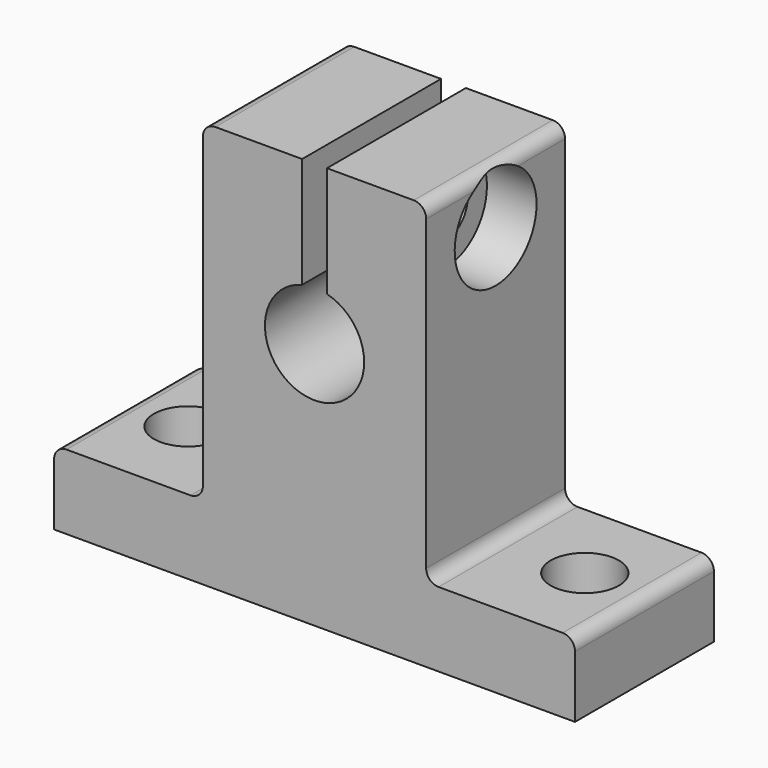
from build123d import *

# Parameters (mm, degrees)
F1_DEPTH       = 14
F3_D           = 4.4
F3_CBORE_D     = 8.25
F3_CBORE_DEPTH = 4
F4_T1_DEPTH    = 14
F4_T3_DEPTH    = 19
F6_D           = 5.5


# Not quite as in the source:
# - a fillet or chamfer that OpenCascade refuses, or shapes differently, is made with other operations: its cross-section is extruded or revolved along the edge and cut away or added


with BuildPart() as f1:
    # F0 (on Front) → F1 (new body)
    with BuildSketch(Plane.XZ):
        with BuildLine():
            Line((-21, 6), (-21, 0))
            Line((-21, 0), (21, 0))
            Line((21, 0), (21, 6))
            Line((21, 6), (9, 6))
            Line((9, 6), (9, 32.8))
            Line((9, 32.8), (1, 32.8))
            Line((1, 32.8), (1, 23.8729833462))
            ThreePointArc((1, 23.8729833462), (3.1622776602, 22.4494897428), (4, 20))
            ThreePointArc((4, 20), (-2.4494897428, 16.8377223398), (-1, 23.8729833462))
            Line((-1, 23.8729833462), (-1, 32.8))
            Line((-1, 32.8), (-9, 32.8))
            Line((-9, 32.8), (-9, 6))
            Line((-9, 6), (-21, 6))
        make_face()
    extrude(amount=F1_DEPTH)

    # F3 (through all)
    with Locations(Plane.YZ.offset(9)):
        with Locations((-7, 28.3364916731)):
            CounterBoreHole(F3_D / 2, F3_CBORE_D / 2, F3_CBORE_DEPTH)

    # F4: fillet of radius 1 on 6 edges, made by hand

    # F4_s2 → F4_t1 (join)
    with BuildSketch(Plane.XZ):
        with BuildLine():
            ThreePointArc((10, 6), (9.2928932188, 6.2928932188), (9, 7))
            Line((9, 7), (9, 6))
            Line((9, 6), (10, 6))
        make_face()
        with BuildLine():
            ThreePointArc((-9, 7), (-9.2928932188, 6.2928932188), (-10, 6))
            Line((-10, 6), (-9, 6))
            Line((-9, 6), (-9, 7))
        make_face()
    extrude(amount=F4_T1_DEPTH)

    # F4_s4 → F4_t3 (cut)
    with BuildSketch(Plane.XZ.offset(-2.5)):
        with BuildLine():
            ThreePointArc((-20, 6), (-20.7071067812, 5.7071067812), (-21, 5))
            Line((-21, 5), (-21, 6))
            Line((-21, 6), (-20, 6))
        make_face()
        with BuildLine():
            ThreePointArc((21, 5), (20.7071067812, 5.7071067812), (20, 6))
            Line((20, 6), (21, 6))
            Line((21, 6), (21, 5))
        make_face()
        with BuildLine():
            ThreePointArc((-8, 32.8), (-8.7071067812, 32.5071067812), (-9, 31.8))
            Line((-9, 31.8), (-9, 32.8))
            Line((-9, 32.8), (-8, 32.8))
        make_face()
        with BuildLine():
            ThreePointArc((9, 31.8), (8.7071067812, 32.5071067812), (8, 32.8))
            Line((8, 32.8), (9, 32.8))
            Line((9, 32.8), (9, 31.8))
        make_face()
    extrude(amount=F4_T3_DEPTH, mode=Mode.SUBTRACT)

    # F6 (through all)
    with Locations(Plane.XY.offset(6)):
        with Locations((-16, -6.7585341167), (16, -6.7585341167)):
            Hole(F6_D / 2)


solid = f1.part
